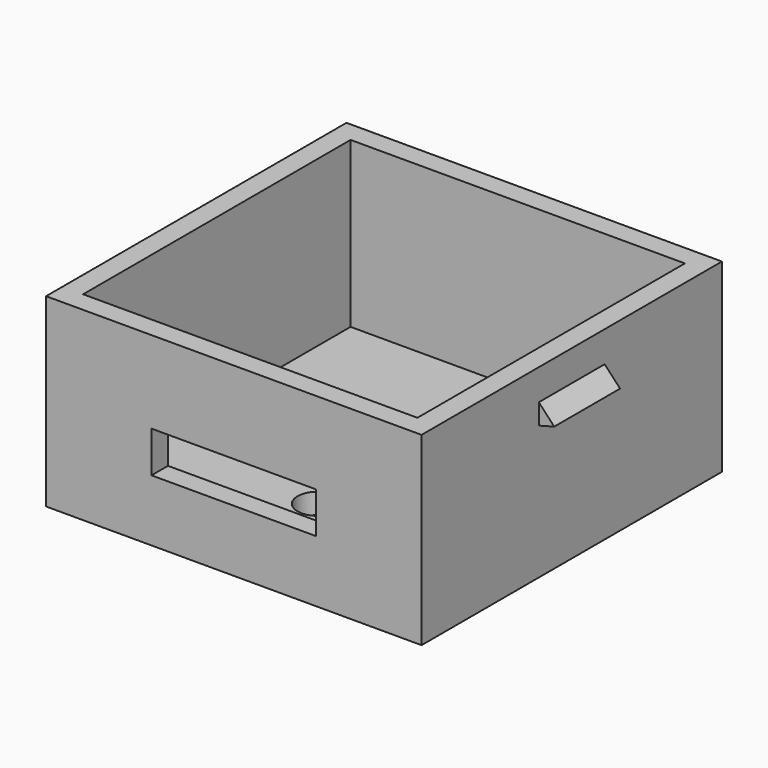
from build123d import *

# Parameters (mm, degrees)
F0_W      = 28.971875
F0_H      = 28.971875
F0_W_2    = 25.796875
F0_H_2    = 25.796875
F1_DEPTH  = 14.2875
F2_W      = 25.796875
F2_H      = 25.796875
F3_DEPTH  = 1.5875
F6_DEPTH  = 3.175
F8_R      = 1.5875
F9_DEPTH  = 1.5885
F10_W     = 12.7
F10_H     = 3.175
F11_DEPTH = 1.5875


# Not quite as in the source:
# - a pattern or mirror of a feature is missing from the dataset's text; its kind, count and spacing are read off the source's solid


with BuildPart() as f1:
    # F0 (on Top) → F1 (new body)
    with BuildSketch(Plane.XY):
        Rectangle(F0_W, F0_H)
        Rectangle(F0_W_2, F0_H_2, mode=Mode.SUBTRACT)
    extrude(amount=F1_DEPTH)

    # F2 (on face) → F3 (join)
    with BuildSketch(Plane(origin=(0, 0, 0), x_dir=(1, 0, 0), z_dir=(0, 0, -1))):
        Rectangle(F2_W, F2_H)
    extrude(amount=-F3_DEPTH)

    # F4: union 

    # F5 (on Front) → F6 (join, symmetric)
    with BuildSketch(Plane.XZ):
        Polygon((14.4859375, 11.90625), (14.4859375, 10.31875), (15.6765625, 10.6377770072), align=None)
    f6 = extrude(amount=F6_DEPTH, both=True)

    # F6_copies: F6 across plane
    add(f6.mirror(Plane(origin=(0, 0, 0), x_dir=(0, 0, -1), z_dir=(-1, 0, 0))))

    # F8 (on face) → F9 (cut, through all)
    with BuildSketch(Plane.XY.offset(1.5875)):
        with Locations((0, 6.35)):
            Circle(F8_R)
        with Locations((0, -6.35)):
            Circle(F8_R)
    extrude(amount=-F9_DEPTH, mode=Mode.SUBTRACT)

    # F10 (on face) → F11 (cut, through all)
    with BuildSketch(Plane.XZ.offset(14.4859375)):
        with Locations((0, 6.35)):
            Rectangle(F10_W, F10_H)
    extrude(amount=-F11_DEPTH, mode=Mode.SUBTRACT)


solid = f1.part
